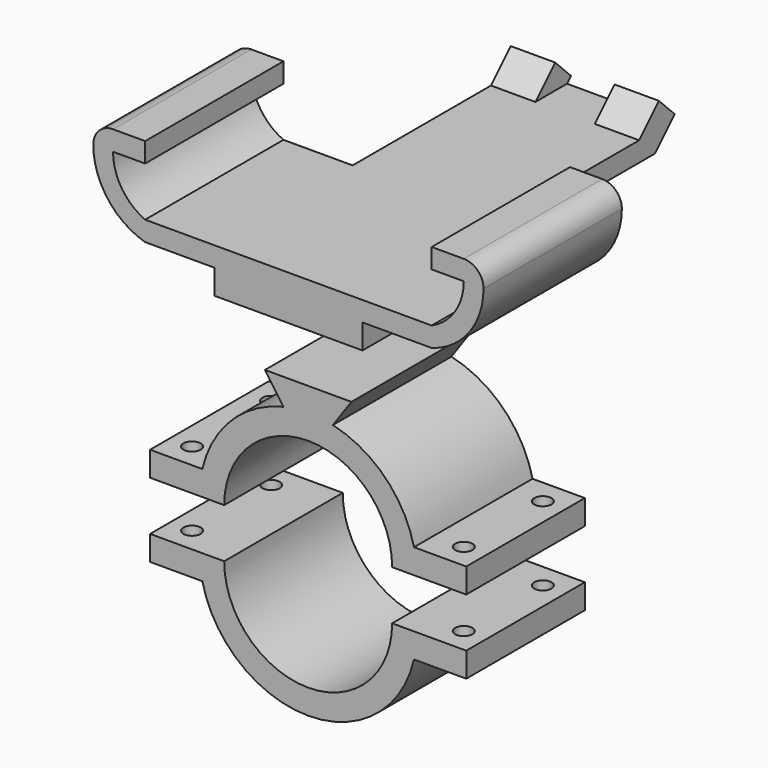
from build123d import *

# Parameters (mm, degrees)
F3_DEPTH      = 30
F4_DEPTH      = 5
F6_DEPTH      = 15
F6_DEPTH_BACK = 15
F7_DEPTH      = 6
F8_DEPTH      = 30
F9_DEPTH      = 30
F10_R         = 1.75
F11_DEPTH     = 50


# Not quite as in the source:
# - a feature names something its author has since deleted; it is built from what else it names


with BuildPart() as f3:
    # F2 (on offset) → F3 (new body)
    with BuildSketch(Plane.XZ.offset(30)):
        with BuildLine():
            Line((29, 49), (-29, 49))
            ThreePointArc((-29, 49), (-33.7322003399, 53.0365697791), (-35.5, 59))
            Line((-35.5, 59), (-29, 59))
            Line((-29, 59), (-29, 63))
            Line((-29, 63), (-35.5, 63))
            ThreePointArc((-35.5, 63), (-38.3284271247, 61.8284271247), (-39.5, 59))
            ThreePointArc((-39.5, 59), (-36.5833333333, 50.25), (-29, 45))
            Line((-29, 45), (-15, 45))
            Line((-15, 45), (-15, 40))
            Line((-15, 40), (-5.748962309, 40))
            Line((-5.748962309, 40), (-9.25, 45))
            Line((-9.25, 45), (9.25, 45))
            Line((9.25, 45), (5.748962309, 40))
            Line((5.748962309, 40), (15, 40))
            Line((15, 40), (15, 45))
            Line((15, 45), (29, 45))
            ThreePointArc((29, 45), (36.5833333333, 50.25), (39.5, 59))
            ThreePointArc((39.5, 59), (38.3284271247, 61.8284271247), (35.5, 63))
            Line((35.5, 63), (29, 63))
            Line((29, 63), (29, 59))
            Line((29, 59), (35.5, 59))
            ThreePointArc((35.5, 59), (33.7322003399, 53.0365697791), (29, 49))
        make_face()
    extrude(amount=-F3_DEPTH)

    # F2 (on offset) → F4 (join)
    with BuildSketch(Plane.XZ.offset(30)):
        with BuildLine():
            Line((29, 49), (-29, 49))
            ThreePointArc((-29, 49), (-33.7322003399, 53.0365697791), (-35.5, 59))
            Line((-35.5, 59), (-29, 59))
            Line((-29, 59), (-29, 63))
            Line((-29, 63), (-35.5, 63))
            ThreePointArc((-35.5, 63), (-38.3284271247, 61.8284271247), (-39.5, 59))
            ThreePointArc((-39.5, 59), (-36.5833333333, 50.25), (-29, 45))
            Line((-29, 45), (-15, 45))
            Line((-15, 45), (-15, 40))
            Line((-15, 40), (-5.748962309, 40))
            Line((-5.748962309, 40), (-9.25, 45))
            Line((-9.25, 45), (9.25, 45))
            Line((9.25, 45), (5.748962309, 40))
            Line((5.748962309, 40), (15, 40))
            Line((15, 40), (15, 45))
            Line((15, 45), (29, 45))
            ThreePointArc((29, 45), (36.5833333333, 50.25), (39.5, 59))
            ThreePointArc((39.5, 59), (38.3284271247, 61.8284271247), (35.5, 63))
            Line((35.5, 63), (29, 63))
            Line((29, 63), (29, 59))
            Line((29, 59), (35.5, 59))
            ThreePointArc((35.5, 59), (33.7322003399, 53.0365697791), (29, 49))
        make_face()
        Polygon((-9.25, 45), (-5.748962309, 40), (5.748962309, 40), (9.25, 45), align=None)
    extrude(amount=F4_DEPTH)

    # F5 (on Right) → F6 (join, two sides)
    with BuildSketch(Plane.YZ) as f6_sk:
        Polygon((35, 49), (0, 49), (0, 45), (39, 45), (43, 49), align=None)
        Polygon((40, 54), (35, 49), (43, 49), (44, 50), align=None)
    extrude(amount=F6_DEPTH)
    extrude(f6_sk.sketch, amount=-F6_DEPTH_BACK)

    # F5 (on Right) → F7 (cut, symmetric)
    with BuildSketch(Plane.YZ):
        Polygon((40, 54), (35, 49), (43, 49), (44, 50), align=None)
    extrude(amount=F7_DEPTH, both=True, mode=Mode.SUBTRACT)


with BuildPart() as f8:
    # F0 (on Front) → F8 (new body)
    with BuildSketch(Plane.XZ):
        with BuildLine():
            Line((-32, 0), (-22, 0))
            ThreePointArc((-22, 0), (-21.8555974099, 2.516517804), (-21.4242852856, 5))
            Line((-21.4242852856, 5), (-32, 5))
            Line((-32, 5), (-32, 0))
        make_face()
        with BuildLine():
            Line((-22, 0), (-17, 0))
            Line((-17, 0), (-17, 5))
            Line((-17, 5), (-21.4242852856, 5))
            ThreePointArc((-21.4242852856, 5), (-21.8555974099, 2.516517804), (-22, 0))
        make_face()
        with BuildLine():
            ThreePointArc((-17, 0), (0, 17), (17, 0))
            Line((17, 0), (17, 5))
            Line((17, 5), (21.4242852856, 5))
            ThreePointArc((21.4242852856, 5), (15.5563491861, 15.5563491861), (5, 21.4242852856))
            ThreePointArc((5, 21.4242852856), (0, 22), (-5, 21.4242852856))
            ThreePointArc((-5, 21.4242852856), (-15.5563491861, 15.5563491861), (-21.4242852856, 5))
            Line((-21.4242852856, 5), (-17, 5))
            Line((-17, 5), (-17, 0))
        make_face()
        with BuildLine():
            Line((17, 5), (17, 0))
            Line((17, 0), (22, 0))
            ThreePointArc((22, 0), (21.8555974099, 2.516517804), (21.4242852856, 5))
            Line((21.4242852856, 5), (17, 5))
        make_face()
        with BuildLine():
            ThreePointArc((21.4242852856, 5), (21.8555974099, 2.516517804), (22, 0))
            Line((22, 0), (32, 0))
            Line((32, 0), (32, 5))
            Line((32, 5), (21.4242852856, 5))
        make_face()
        with BuildLine():
            ThreePointArc((-5, 21.4242852856), (0, 22), (5, 21.4242852856))
            Line((5, 21.4242852856), (8.75, 26.7798403109))
            Line((8.75, 26.7798403109), (-8.75, 26.7798403109))
            Line((-8.75, 26.7798403109), (-5, 21.4242852856))
        make_face()
    extrude(amount=F8_DEPTH)


with BuildPart() as f9:
    # F0 (on Front) → F9 (new body)
    with BuildSketch(Plane.XZ):
        with BuildLine():
            ThreePointArc((-21.4242852856, -15), (-21.8555974099, -12.516517804), (-22, -10))
            Line((-22, -10), (-32, -10))
            Line((-32, -10), (-32, -15))
            Line((-32, -15), (-21.4242852856, -15))
        make_face()
        with BuildLine():
            Line((-17, -15), (-17, -10))
            Line((-17, -10), (-22, -10))
            ThreePointArc((-22, -10), (-21.8555974099, -12.516517804), (-21.4242852856, -15))
            Line((-21.4242852856, -15), (-17, -15))
        make_face()
        with BuildLine():
            ThreePointArc((17, -10), (0, -27), (-17, -10))
            Line((-17, -10), (-17, -15))
            Line((-17, -15), (-21.4242852856, -15))
            ThreePointArc((-21.4242852856, -15), (0, -32), (21.4242852856, -15))
            Line((21.4242852856, -15), (17, -15))
            Line((17, -15), (17, -10))
        make_face()
        with BuildLine():
            Line((22, -10), (17, -10))
            Line((17, -10), (17, -15))
            Line((17, -15), (21.4242852856, -15))
            ThreePointArc((21.4242852856, -15), (21.8555974099, -12.516517804), (22, -10))
        make_face()
        with BuildLine():
            Line((32, -10), (22, -10))
            ThreePointArc((22, -10), (21.8555974099, -12.516517804), (21.4242852856, -15))
            Line((21.4242852856, -15), (32, -15))
            Line((32, -15), (32, -10))
        make_face()
    extrude(amount=F9_DEPTH)


with BuildPart() as f11_tool:
    # F10 (on face) → F11 (new body)
    with BuildSketch(Plane.XY.offset(5)):
        with Locations((-27.5, -25)):
            Circle(F10_R)
        with Locations((-27.5, -5)):
            Circle(F10_R)
        with Locations((27.5, -5)):
            Circle(F10_R)
        with Locations((27.5, -25)):
            Circle(F10_R)
    extrude(amount=-F11_DEPTH)


with BuildPart() as f8_1:
    add(f8.part)

    # F11: cut by f11_tool
    add(f11_tool.part, mode=Mode.SUBTRACT)


with BuildPart() as f9_1:
    add(f9.part)

    # F11: cut by f11_tool
    add(f11_tool.part, mode=Mode.SUBTRACT)


solid = Compound([f3.part, f8_1.part, f9_1.part])
